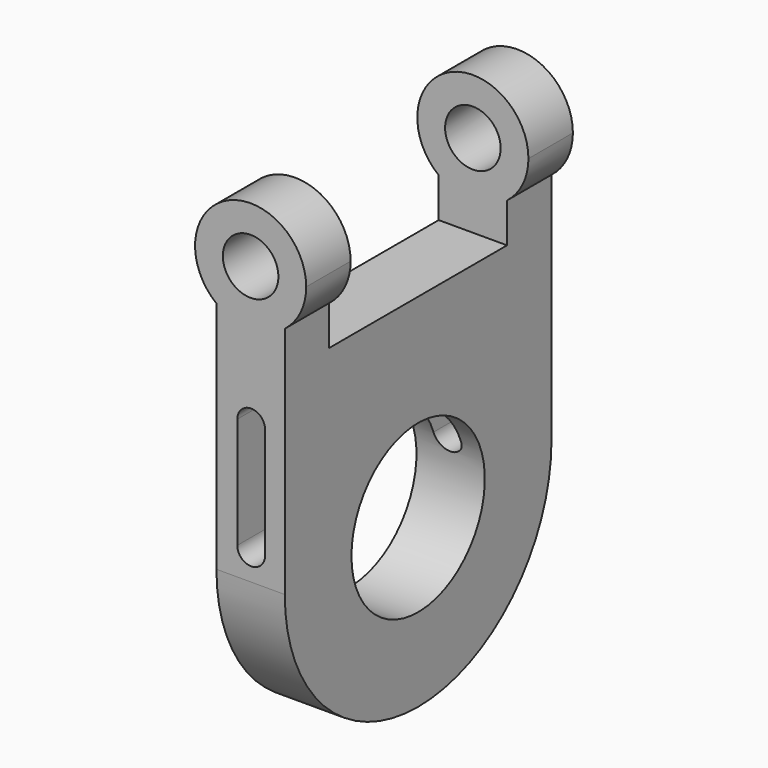
from build123d import *

# Parameters (mm, degrees)
F0_R          = 12.7
F1_DEPTH      = 152.4
F2_R          = 76.19999
F3_W          = 101.6
F3_H          = 56.6531687857
F4_DEPTH      = 41.022
F4_DEPTH_BACK = 25.4
F6_DEPTH      = 152.401
F3_H_2        = 18.0714114576
F7_DEPTH      = 41.022
F3_R          = 38.1
F8_DEPTH      = 41.022


# Not quite as in the source:
# - a fillet or chamfer is up to 0.001 mm smaller than in the source, because OpenCascade refuses the exact size
# - a feature names something its author has since deleted; it is built from what else it names


with BuildPart() as f1:
    # F0 (on Front) → F1 (new body)
    with BuildSketch(Plane.XZ):
        with BuildLine():
            ThreePointArc((15.621, 18.2628701244), (22.8246949596, 27.1472538948), (25.4, 38.2914586668))
            ThreePointArc((25.4, 38.2914586668), (-11.144204772, 61.1161536264), (-15.621, 18.2628701244))
            ThreePointArc((-15.621, 18.2628701244), (0, 12.8914586668), (15.621, 18.2628701244))
        make_face()
        with Locations((0, 38.2914586668)):
            Circle(F0_R, mode=Mode.SUBTRACT)
        with BuildLine():
            ThreePointArc((15.621, 18.2628701244), (0, 12.8914586668), (-15.621, 18.2628701244))
            Line((-15.621, 18.2628701244), (-15.621, -164.9085413332))
            Line((-15.621, -164.9085413332), (15.621, -164.9085413332))
            Line((15.621, -164.9085413332), (15.621, 18.2628701244))
        make_face()
    extrude(amount=F1_DEPTH)

    # F2 (radius 76.2 in the source; OpenCascade refuses exactly that, so slightly less here)
    f2_edges = [f1.edges().sort_by_distance(p)[0] for p in [
        (0, -152.4, -164.908541),
        (0, 0, -164.908541),
    ]]
    fillet(f2_edges, radius=F2_R)

    # F3 (on face) → F4 (cut, two sides)
    with BuildSketch(Plane(origin=(-15.621, 0, 0), x_dir=(0, -1, 0), z_dir=(-1, 0, 0))) as f4_sk:
        with Locations((76.2, 46.5894545172)):
            Rectangle(F3_W, F3_H)
    extrude(amount=-F4_DEPTH, mode=Mode.SUBTRACT)
    extrude(f4_sk.sketch, amount=F4_DEPTH_BACK, mode=Mode.SUBTRACT)

    # F5 (on Front) → F6 (cut, through all)
    with BuildSketch(Plane.XZ):
        with BuildLine():
            ThreePointArc((6.604, -25.2085413332), (0.254, -18.8585413332), (-6.096, -25.2085413332))
            Line((-6.096, -25.2085413332), (-6.096, -76.0085413332))
            ThreePointArc((-6.096, -76.0085413332), (0.254, -82.3585413332), (6.604, -76.0085413332))
            Line((6.604, -76.0085413332), (6.604, -25.2085413332))
        make_face()
    extrude(amount=F6_DEPTH, mode=Mode.SUBTRACT)

    # F3 (on face) → F7 (cut, through all)
    with BuildSketch(Plane(origin=(-15.621, 0, 0), x_dir=(0, -1, 0), z_dir=(-1, 0, 0))):
        with Locations((76.2, 9.2271643956)):
            Rectangle(F3_W, F3_H_2)
    extrude(amount=-F7_DEPTH, mode=Mode.SUBTRACT)

    # F3 (on face) → F8 (cut, through all)
    with BuildSketch(Plane(origin=(-15.621, 0, 0), x_dir=(0, -1, 0), z_dir=(-1, 0, 0))):
        with Locations((76.2, -88.7085413332)):
            Circle(F3_R)
    extrude(amount=-F8_DEPTH, mode=Mode.SUBTRACT)


solid = f1.part
